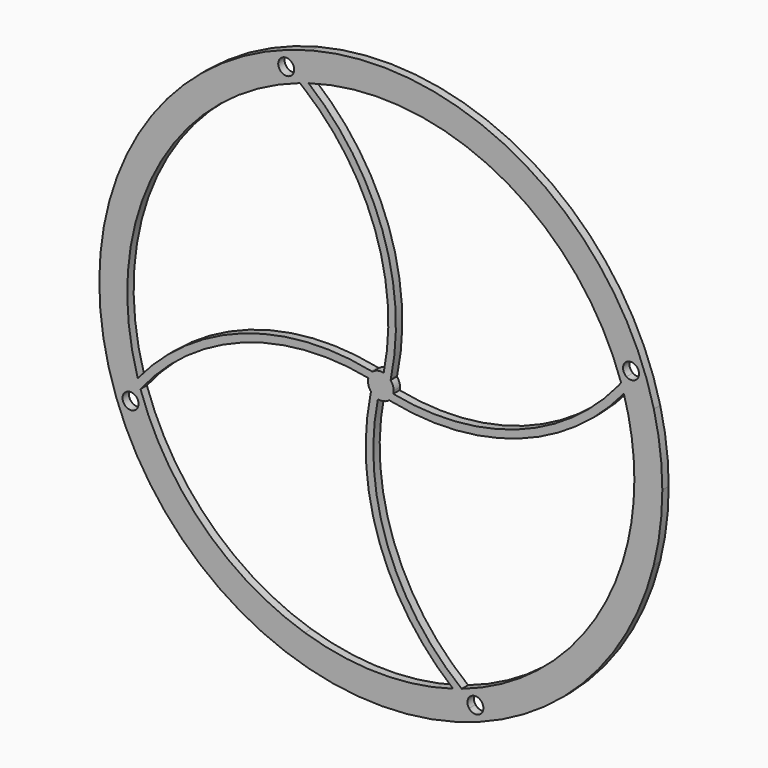
from build123d import *

# Parameters (mm, degrees)
F1_DEPTH = 2


# Not quite as in the source:
# - a feature names something its author has since deleted; it is built from what else it names


with BuildPart() as f1:
    # F0 (on Front) → F1 (new body)
    with BuildSketch(Plane.XZ):
        with BuildLine():
            ThreePointArc((-27.3670955133, 56.9056551345), (-80.5728095325, -11.5155179666), (-27.2210675465, -79.822886236))
            ThreePointArc((-27.2210675465, -79.822886236), (-28.2707166424, -75.9512965825), (-29.0922663621, -72.0249718726))
            ThreePointArc((-29.0922663621, -72.0249718726), (-54.5082769695, -56.802573142), (-70.2520814599, -31.7062061045))
            ThreePointArc((-70.2520814599, -31.7062061045), (-70.6313699985, -32.1947433172), (-71.0054179832, -32.6873044899))
            ThreePointArc((-71.0054179832, -32.6873044899), (-70.0780888504, -33.7565825815), (-69.7442063574, -35.1320161272))
            ThreePointArc((-69.7442063574, -35.1320161272), (-74.7859973818, -37.3299900608), (-72.9649326324, -32.1401471609))
            ThreePointArc((-72.9649326324, -32.1401471609), (-71.9713178078, -30.821081237), (-70.9416554734, -29.5299573821))
            ThreePointArc((-70.9416554734, -29.5299573821), (-66.4396950536, 17.8006515976), (-30.3388328071, 48.7390086816))
            ThreePointArc((-30.3388328071, 48.7390086816), (-30.8273700198, 49.1182972202), (-31.3199311925, 49.4923452049))
            ThreePointArc((-31.3199311925, 49.4923452049), (-36.6541110474, 52.0379628175), (-30.7727738636, 51.4518598542))
            ThreePointArc((-30.7727738636, 51.4518598542), (-29.8904735112, 50.7935939017), (-29.0204405195, 50.1191974536))
            ThreePointArc((-29.0204405195, 50.1191974536), (-28.2798956872, 53.5334090749), (-27.3670955133, 56.9056551345))
        make_face()
        with BuildLine():
            ThreePointArc((-29.0922663621, -72.0249718726), (-28.2707166424, -75.9512965825), (-27.2210675465, -79.822886236))
            ThreePointArc((-27.2210675465, -79.822886236), (26.0907604983, -71.958346724), (58.2730284319, -28.7344688106))
            ThreePointArc((58.2730284319, -28.7344688106), (54.4014575958, -29.7669456779), (50.4763758376, -30.5724283969))
            ThreePointArc((50.4763758376, -30.5724283969), (35.2481065637, -55.9178682056), (10.1931333262, -71.6194547573))
            ThreePointArc((10.1931333262, -71.6194547573), (10.6816705389, -71.9987432958), (11.1742317116, -72.3727912805))
            ThreePointArc((11.1742317116, -72.3727912805), (14.5315947304, -71.2537714989), (16.6189433489, -74.1115796548))
            ThreePointArc((16.6189433489, -74.1115796548), (13.7293813431, -77.1095462072), (10.6270743826, -74.3323059298))
            ThreePointArc((10.6270743826, -74.3323059298), (9.3080084587, -73.3386911051), (8.0168846038, -72.3090287708))
            ThreePointArc((8.0168846038, -72.3090287708), (-10.5589046392, -74.9383627794), (-29.0922663621, -72.0249718726))
        make_face()
        with BuildLine():
            ThreePointArc((58.3098134577, 5.7079947682), (26.0907604983, 49.0779006484), (-27.3670955133, 56.9056551345))
            ThreePointArc((-27.3670955133, 56.9056551345), (-28.2798956872, 53.5334090749), (-29.0204405195, 50.1191974536))
            ThreePointArc((-29.0204405195, 50.1191974536), (-28.589922312, 49.7758651019), (-28.1625840847, 49.4285826951))
            ThreePointArc((-28.1625840847, 49.4285826951), (19.1680248949, 44.9266222753), (50.106381979, 8.8257600288))
            ThreePointArc((50.106381979, 8.8257600288), (50.4856705176, 9.3142972415), (50.8597185023, 9.8068584143))
            ThreePointArc((50.8597185023, 9.8068584143), (51.2230733308, 14.9176875586), (55.5985068765, 12.2515700516))
            ThreePointArc((55.5985068765, 12.2515700516), (54.79648081, 10.2097790271), (52.8192331515, 9.2597010853))
            ThreePointArc((52.8192331515, 9.2597010853), (52.1241754763, 8.329073827), (51.4111721259, 7.4121231804))
            ThreePointArc((51.4111721259, 7.4121231804), (54.8825742735, 6.6494490821), (58.3098134577, 5.7079947682))
        make_face()
        with BuildLine():
            ThreePointArc((50.4763758376, -30.5724283969), (54.4014575958, -29.7669456779), (58.2730284319, -28.7344688106))
            ThreePointArc((58.2730284319, -28.7344688106), (59.886547095, -20.1541655683), (60.4271502595, -11.4402230378))
            ThreePointArc((60.4271502595, -11.4402230378), (59.8958138007, -2.8010030346), (58.3098134577, 5.7079947682))
            ThreePointArc((58.3098134577, 5.7079947682), (54.8825742735, 6.6494490821), (51.4111721259, 7.4121231804))
            ThreePointArc((51.4111721259, 7.4121231804), (51.1051261442, 7.0295570743), (50.7959559925, 6.6495113064))
            ThreePointArc((50.7959559925, 6.6495113064), (52.7659088566, -2.3001782907), (53.4271502595, -11.4402230378))
            ThreePointArc((53.4271502595, -11.4402230378), (52.6851211645, -21.1194320912), (50.4763758376, -30.5724283969))
        make_face()
        with BuildLine():
            ThreePointArc((-12.5201116119, -13.51897209), (-12.5889413468, -13.8437334785), (-12.6559669985, -14.1688719933))
            ThreePointArc((-12.6559669985, -14.1688719933), (-12.4731783685, -13.96568891), (-12.2895816621, -13.7632357104))
            ThreePointArc((-12.2895816621, -13.7632357104), (-12.4080426029, -13.6441201736), (-12.5201116119, -13.51897209))
        make_face()
        with BuildLine():
            ThreePointArc((-12.2895816621, -13.7632357104), (-12.4731783685, -13.96568891), (-12.6559669985, -14.1688719933))
            ThreePointArc((-12.6559669985, -14.1688719933), (-10.3985570941, -46.1115999582), (8.0168846038, -72.3090287708))
            ThreePointArc((8.0168846038, -72.3090287708), (9.1081080721, -71.9740223354), (10.1931333262, -71.6194547573))
            ThreePointArc((10.1931333262, -71.6194547573), (-8.3929341527, -46.0705747238), (-10.7982724135, -14.5681696862))
            ThreePointArc((-10.7982724135, -14.5681696862), (-11.5979884526, -14.2658628235), (-12.2895816621, -13.7632357104))
        make_face()
        with BuildLine():
            ThreePointArc((-70.9416554734, -29.5299573821), (-70.606649038, -30.6211808503), (-70.2520814599, -31.7062061045))
            ThreePointArc((-70.2520814599, -31.7062061045), (-44.7032014264, -13.1201386255), (-13.2007963888, -10.7148003648))
            ThreePointArc((-13.2007963888, -10.7148003648), (-12.862086438, -9.8494851792), (-12.2897757069, -9.1173955477))
            ThreePointArc((-12.2897757069, -9.1173955477), (-12.3762338407, -9.022292149), (-12.4625142647, -8.9270274978))
            ThreePointArc((-12.4625142647, -8.9270274978), (-44.5810834921, -11.0567727884), (-70.9416554734, -29.5299573821))
        make_face()
        with BuildLine():
            ThreePointArc((-71.0054179832, -32.6873044899), (-70.6313699985, -32.1947433172), (-70.2520814599, -31.7062061045))
            ThreePointArc((-70.2520814599, -31.7062061045), (-70.606649038, -30.6211808503), (-70.9416554734, -29.5299573821))
            ThreePointArc((-70.9416554734, -29.5299573821), (-71.9713178078, -30.821081237), (-72.9649326324, -32.1401471609))
            ThreePointArc((-72.9649326324, -32.1401471609), (-71.937377119, -32.2425479097), (-71.0054179832, -32.6873044899))
        make_face()
        with BuildLine():
            ThreePointArc((10.1931333262, -71.6194547573), (9.1081080721, -71.9740223354), (8.0168846038, -72.3090287708))
            ThreePointArc((8.0168846038, -72.3090287708), (9.3080084587, -73.3386911051), (10.6270743826, -74.3323059298))
            ThreePointArc((10.6270743826, -74.3323059298), (10.7294751314, -73.3047504164), (11.1742317116, -72.3727912805))
            ThreePointArc((11.1742317116, -72.3727912805), (10.6816705389, -71.9987432958), (10.1931333262, -71.6194547573))
        make_face()
        with BuildLine():
            ThreePointArc((-28.1625840847, 49.4285826951), (-28.589922312, 49.7758651019), (-29.0204405195, 50.1191974536))
            ThreePointArc((-29.0204405195, 50.1191974536), (-29.1146314874, 49.6144442417), (-29.2050550996, 49.1090025402))
            ThreePointArc((-29.2050550996, 49.1090025402), (-28.6845055424, 49.2710301885), (-28.1625840847, 49.4285826951))
        make_face()
        with BuildLine():
            ThreePointArc((-29.2050550996, 49.1090025402), (-29.1146314874, 49.6144442417), (-29.0204405195, 50.1191974536))
            ThreePointArc((-29.0204405195, 50.1191974536), (-29.8904735112, 50.7935939017), (-30.7727738636, 51.4518598542))
            ThreePointArc((-30.7727738636, 51.4518598542), (-30.7666762774, 51.3415715733), (-30.7646428299, 51.2311335791))
            ThreePointArc((-30.7646428299, 51.2311335791), (-30.9068346739, 50.3184821977), (-31.3199311925, 49.4923452049))
            ThreePointArc((-31.3199311925, 49.4923452049), (-30.8273700198, 49.1182972202), (-30.3388328071, 48.7390086816))
            ThreePointArc((-30.3388328071, 48.7390086816), (-29.7728126001, 48.9266674182), (-29.2050550996, 49.1090025402))
        make_face()
        with BuildLine():
            ThreePointArc((50.7959559925, 6.6495113064), (51.1051261442, 7.0295570743), (51.4111721259, 7.4121231804))
            ThreePointArc((51.4111721259, 7.4121231804), (50.9618140768, 7.4971572567), (50.5118990943, 7.5791935838))
            ThreePointArc((50.5118990943, 7.5791935838), (50.6557066113, 7.1148960249), (50.7959559925, 6.6495113064))
        make_face()
        with BuildLine():
            ThreePointArc((50.5118990943, 7.5791935838), (50.9618140768, 7.4971572567), (51.4111721259, 7.4121231804))
            ThreePointArc((51.4111721259, 7.4121231804), (52.1241754763, 8.329073827), (52.8192331515, 9.2597010853))
            ThreePointArc((52.8192331515, 9.2597010853), (51.7916776381, 9.362101834), (50.8597185023, 9.8068584143))
            ThreePointArc((50.8597185023, 9.8068584143), (50.4856705176, 9.3142972415), (50.106381979, 8.8257600288))
            ThreePointArc((50.106381979, 8.8257600288), (50.3123573205, 8.2035232495), (50.5118990943, 7.5791935838))
        make_face()
        with BuildLine():
            ThreePointArc((-12.5201116119, -13.51897209), (-12.4080426029, -13.6441201736), (-12.2895816621, -13.7632357104))
            ThreePointArc((-12.2895816621, -13.7632357104), (-11.1948099524, -12.5887570771), (-10.0728497405, -11.4402230378))
            ThreePointArc((-10.0728497405, -11.4402230378), (-10.9940718567, -11.2075300608), (-11.9189886514, -10.9899866588))
            ThreePointArc((-11.9189886514, -10.9899866588), (-12.2332943861, -12.2512124569), (-12.5201116119, -13.51897209))
        make_face()
        with BuildLine():
            ThreePointArc((-10.0728497405, -11.4402230378), (-11.1948099524, -12.5887570771), (-12.2895816621, -13.7632357104))
            ThreePointArc((-12.2895816621, -13.7632357104), (-11.5979884526, -14.2658628235), (-10.7982724135, -14.5681696862))
            ThreePointArc((-10.7982724135, -14.5681696862), (-10.6643076305, -13.9264868582), (-10.5230861195, -13.2863619488))
            ThreePointArc((-10.5230861195, -13.2863619488), (-10.5381735464, -13.2824253135), (-10.5532599463, -13.2784847442))
            Line((-10.5532599463, -13.2784847442), (-10.0728497405, -11.4402230378))
        make_face()
        with BuildLine():
            ThreePointArc((-13.2007963888, -10.7148003648), (-13.1931994446, -12.1976568722), (-12.5201116119, -13.51897209))
            ThreePointArc((-12.5201116119, -13.51897209), (-12.2332943861, -12.2512124569), (-11.9189886514, -10.9899866588))
            ThreePointArc((-11.9189886514, -10.9899866588), (-12.5591135608, -10.8487651478), (-13.2007963888, -10.7148003648))
        make_face()
        with BuildLine():
            ThreePointArc((-12.2897757069, -9.1173955477), (-12.862086438, -9.8494851792), (-13.2007963888, -10.7148003648))
            ThreePointArc((-13.2007963888, -10.7148003648), (-12.5591135608, -10.8487651478), (-11.9189886514, -10.9899866588))
            ThreePointArc((-11.9189886514, -10.9899866588), (-11.9150520162, -10.9748992319), (-11.9111114468, -10.9598128319))
            Line((-11.9111114468, -10.9598128319), (-10.0728497405, -11.4402230378))
            ThreePointArc((-10.0728497405, -11.4402230378), (-11.1948573752, -10.2917364213), (-12.2897757069, -9.1173955477))
        make_face()
        with BuildLine():
            ThreePointArc((-69.7442063574, -35.1320161272), (-70.0780888504, -33.7565825815), (-71.0054179832, -32.6873044899))
            ThreePointArc((-71.0054179832, -32.6873044899), (-71.3040153489, -33.088497971), (-71.5991359801, -33.4922558304))
            ThreePointArc((-71.5991359801, -33.4922558304), (-70.9707717301, -34.2073920832), (-70.7442063574, -35.1320161272))
            ThreePointArc((-70.7442063574, -35.1320161272), (-73.6278272269, -36.9262329923), (-73.9634205165, -33.5466086609))
            ThreePointArc((-73.9634205165, -33.5466086609), (-73.469248174, -32.839777435), (-72.9649326324, -32.1401471609))
            ThreePointArc((-72.9649326324, -32.1401471609), (-74.7859973818, -37.3299900608), (-69.7442063574, -35.1320161272))
        make_face()
        with BuildLine():
            ThreePointArc((-71.5991359801, -33.4922558304), (-71.3040153489, -33.088497971), (-71.0054179832, -32.6873044899))
            ThreePointArc((-71.0054179832, -32.6873044899), (-71.937377119, -32.2425479097), (-72.9649326324, -32.1401471609))
            ThreePointArc((-72.9649326324, -32.1401471609), (-73.469248174, -32.839777435), (-73.9634205165, -33.5466086609))
            ThreePointArc((-73.9634205165, -33.5466086609), (-72.7901724606, -33.1325444177), (-71.5991359801, -33.4922558304))
        make_face()
        with BuildLine():
            ThreePointArc((11.1742317116, -72.3727912805), (10.7294751314, -73.3047504164), (10.6270743826, -74.3323059298))
            ThreePointArc((10.6270743826, -74.3323059298), (11.3267046567, -74.8366214714), (12.0335358826, -75.3307938138))
            ThreePointArc((12.0335358826, -75.3307938138), (11.6194716394, -74.1575457579), (11.9791830521, -72.9665092775))
            ThreePointArc((11.9791830521, -72.9665092775), (11.5754251927, -72.6713886463), (11.1742317116, -72.3727912805))
        make_face()
        with BuildLine():
            ThreePointArc((12.0335358826, -75.3307938138), (11.3267046567, -74.8366214714), (10.6270743826, -74.3323059298))
            ThreePointArc((10.6270743826, -74.3323059298), (13.7293813431, -77.1095462072), (16.6189433489, -74.1115796548))
            ThreePointArc((16.6189433489, -74.1115796548), (14.5315947304, -71.2537714989), (11.1742317116, -72.3727912805))
            ThreePointArc((11.1742317116, -72.3727912805), (11.5754251927, -72.6713886463), (11.9791830521, -72.9665092775))
            ThreePointArc((11.9791830521, -72.9665092775), (14.2191430683, -72.2037640723), (15.6189433489, -74.1115796548))
            ThreePointArc((15.6189433489, -74.1115796548), (14.2628319524, -76.0050968758), (12.0335358826, -75.3307938138))
        make_face()
        with BuildLine():
            ThreePointArc((-28.1625840847, 49.4285826951), (-28.6845055424, 49.2710301885), (-29.2050550996, 49.1090025402))
            ThreePointArc((-29.2050550996, 49.1090025402), (-29.3013575877, 48.545087408), (-29.3929706411, 47.9803914774))
            ThreePointArc((-29.3929706411, 47.9803914774), (-11.5464019221, 22.6200733478), (-9.3474270674, -8.3122763895))
            ThreePointArc((-9.3474270674, -8.3122763895), (-8.4819953839, -8.6510527838), (-7.7498370678, -9.2234911162))
            ThreePointArc((-7.7498370678, -9.2234911162), (-7.6548806672, -9.1371958925), (-7.5597630163, -9.051078437))
            ThreePointArc((-7.5597630163, -9.051078437), (-9.6893112365, 23.0677602114), (-28.1625840847, 49.4285826951))
        make_face()
        with BuildLine():
            ThreePointArc((-29.3929706411, 47.9803914774), (-29.3013575877, 48.545087408), (-29.2050550996, 49.1090025402))
            ThreePointArc((-29.2050550996, 49.1090025402), (-29.7728126001, 48.9266674182), (-30.3388328071, 48.7390086816))
            ThreePointArc((-30.3388328071, 48.7390086816), (-29.8639157079, 48.3621762923), (-29.3929706411, 47.9803914774))
        make_face()
        with BuildLine():
            ThreePointArc((-30.7646428299, 51.2311335791), (-30.7666762774, 51.3415715733), (-30.7727738636, 51.4518598542))
            ThreePointArc((-30.7727738636, 51.4518598542), (-31.4724041376, 51.9561753958), (-32.1792353635, 52.4503477382))
            ThreePointArc((-32.1792353635, 52.4503477382), (-31.8711256088, 51.8750221826), (-31.7646428299, 51.2311335791))
            ThreePointArc((-31.7646428299, 51.2311335791), (-31.8568272474, 50.6309338597), (-32.124882533, 50.0860632018))
            ThreePointArc((-32.124882533, 50.0860632018), (-31.7211246736, 49.7909425706), (-31.3199311925, 49.4923452049))
            ThreePointArc((-31.3199311925, 49.4923452049), (-30.9068346739, 50.3184821977), (-30.7646428299, 51.2311335791))
        make_face()
        with BuildLine():
            ThreePointArc((-32.1792353635, 52.4503477382), (-31.4724041376, 51.9561753958), (-30.7727738636, 51.4518598542))
            ThreePointArc((-30.7727738636, 51.4518598542), (-36.6541110474, 52.0379628175), (-31.3199311925, 49.4923452049))
            ThreePointArc((-31.3199311925, 49.4923452049), (-31.7211246736, 49.7909425706), (-32.124882533, 50.0860632018))
            ThreePointArc((-32.124882533, 50.0860632018), (-35.7641145394, 51.185167476), (-32.1792353635, 52.4503477382))
        make_face()
        with BuildLine():
            ThreePointArc((-7.9941006882, -13.8874849093), (-7.6696946098, -13.9562403689), (-7.3449122183, -14.0231956907))
            ThreePointArc((-7.3449122183, -14.0231956907), (-7.5478301275, -13.8405739674), (-7.7500222504, -13.6571490043))
            ThreePointArc((-7.7500222504, -13.6571490043), (-7.8690501416, -13.7755079493), (-7.9941006882, -13.8874849093))
        make_face()
        with BuildLine():
            ThreePointArc((-7.7500222504, -13.6571490043), (-7.5478301275, -13.8405739674), (-7.3449122183, -14.0231956907))
            ThreePointArc((-7.3449122183, -14.0231956907), (24.5981851662, -11.7660519999), (50.7959559925, 6.6495113064))
            ThreePointArc((50.7959559925, 6.6495113064), (50.6557066113, 7.1148960249), (50.5118990943, 7.5791935838))
            ThreePointArc((50.5118990943, 7.5791935838), (49.8930363162, 7.6869831447), (49.2732124019, 7.7891009341))
            ThreePointArc((49.2732124019, 7.7891009341), (23.9320992091, -9.9863481746), (-6.9449030921, -12.1656457109))
            ThreePointArc((-6.9449030921, -12.1656457109), (-7.2472736584, -12.9654797683), (-7.7500222504, -13.6571490043))
        make_face()
        with BuildLine():
            ThreePointArc((49.2732124019, 7.7891009341), (49.8930363162, 7.6869831447), (50.5118990943, 7.5791935838))
            ThreePointArc((50.5118990943, 7.5791935838), (50.3123573205, 8.2035232495), (50.106381979, 8.8257600288))
            ThreePointArc((50.106381979, 8.8257600288), (49.6927740639, 8.3050379491), (49.2732124019, 7.7891009341))
        make_face()
        with BuildLine():
            ThreePointArc((50.8597185023, 9.8068584143), (51.7916776381, 9.362101834), (52.8192331515, 9.2597010853))
            ThreePointArc((52.8192331515, 9.2597010853), (53.0275327482, 9.5460981807), (53.2341325227, 9.8337238948))
            ThreePointArc((53.2341325227, 9.8337238948), (52.1548181767, 9.7912569947), (51.1583297131, 10.2080706662))
            ThreePointArc((51.1583297131, 10.2080706662), (51.0094573534, 10.0071420874), (50.8597185023, 9.8068584143))
        make_face()
        with BuildLine():
            ThreePointArc((53.2341325227, 9.8337238948), (53.0275327482, 9.5460981807), (52.8192331515, 9.2597010853))
            ThreePointArc((52.8192331515, 9.2597010853), (54.79648081, 10.2097790271), (55.5985068765, 12.2515700516))
            ThreePointArc((55.5985068765, 12.2515700516), (51.2230733308, 14.9176875586), (50.8597185023, 9.8068584143))
            ThreePointArc((50.8597185023, 9.8068584143), (51.0094573534, 10.0071420874), (51.1583297131, 10.2080706662))
            ThreePointArc((51.1583297131, 10.2080706662), (51.4475166308, 14.4708540474), (55.0985068765, 12.2515700516))
            ThreePointArc((55.0985068765, 12.2515700516), (54.578287687, 10.7249830274), (53.2341325227, 9.8337238948))
        make_face()
        with BuildLine():
            Line((-9.5924395346, -9.6019613315), (-10.0728497405, -11.4402230378))
            ThreePointArc((-10.0728497405, -11.4402230378), (-8.9243157011, -10.3182628259), (-7.7498370678, -9.2234911162))
            ThreePointArc((-7.7498370678, -9.2234911162), (-8.4819953839, -8.6510527838), (-9.3474270674, -8.3122763895))
            ThreePointArc((-9.3474270674, -8.3122763895), (-9.4813918505, -8.9539592174), (-9.6226133615, -9.5940841269))
            ThreePointArc((-9.6226133615, -9.5940841269), (-9.6075259345, -9.5980207621), (-9.5924395346, -9.6019613315))
        make_face()
        with BuildLine():
            Line((-8.2345880341, -11.9206332437), (-10.0728497405, -11.4402230378))
            ThreePointArc((-10.0728497405, -11.4402230378), (-8.924363124, -12.5622306726), (-7.7500222504, -13.6571490043))
            ThreePointArc((-7.7500222504, -13.6571490043), (-7.2472736584, -12.9654797683), (-6.9449030921, -12.1656457109))
            ThreePointArc((-6.9449030921, -12.1656457109), (-7.5865859201, -12.0316809278), (-8.2267108295, -11.8904594168))
            ThreePointArc((-8.2267108295, -11.8904594168), (-8.2306474647, -11.9055468438), (-8.2345880341, -11.9206332437))
        make_face()
        with BuildLine():
            ThreePointArc((-7.7498370678, -9.2234911162), (-8.9243157011, -10.3182628259), (-10.0728497405, -11.4402230378))
            ThreePointArc((-10.0728497405, -11.4402230378), (-9.1516276243, -11.6729160149), (-8.2267108295, -11.8904594168))
            ThreePointArc((-8.2267108295, -11.8904594168), (-7.9124050948, -10.6292336188), (-7.625587869, -9.3614739856))
            ThreePointArc((-7.625587869, -9.3614739856), (-7.686714869, -9.2915842443), (-7.7498370678, -9.2234911162))
        make_face()
        with BuildLine():
            ThreePointArc((-10.5230861195, -13.2863619488), (-10.3055427175, -12.361445154), (-10.0728497405, -11.4402230378))
            Line((-10.0728497405, -11.4402230378), (-10.5532599463, -13.2784847442))
            ThreePointArc((-10.5532599463, -13.2784847442), (-10.5381735464, -13.2824253135), (-10.5230861195, -13.2863619488))
        make_face()
        with BuildLine():
            ThreePointArc((-12.2897757069, -9.1173955477), (-11.1948573752, -10.2917364213), (-10.0728497405, -11.4402230378))
            ThreePointArc((-10.0728497405, -11.4402230378), (-9.8401567634, -10.5190009216), (-9.6226133615, -9.5940841269))
            ThreePointArc((-9.6226133615, -9.5940841269), (-10.8838391595, -9.2797783922), (-12.1515987927, -8.9929611664))
            ThreePointArc((-12.1515987927, -8.9929611664), (-12.2215881949, -9.0541779116), (-12.2897757069, -9.1173955477))
        make_face()
        with BuildLine():
            ThreePointArc((-8.2267108295, -11.8904594168), (-9.1516276243, -11.6729160149), (-10.0728497405, -11.4402230378))
            Line((-10.0728497405, -11.4402230378), (-8.2345880341, -11.9206332437))
            ThreePointArc((-8.2345880341, -11.9206332437), (-8.2306474647, -11.9055468438), (-8.2267108295, -11.8904594168))
        make_face()
        with BuildLine():
            ThreePointArc((-9.6226133615, -9.5940841269), (-9.8401567634, -10.5190009216), (-10.0728497405, -11.4402230378))
            Line((-10.0728497405, -11.4402230378), (-9.5924395346, -9.6019613315))
            ThreePointArc((-9.5924395346, -9.6019613315), (-9.6075259345, -9.5980207621), (-9.6226133615, -9.5940841269))
        make_face()
        with BuildLine():
            ThreePointArc((-7.7500222504, -13.6571490043), (-8.924363124, -12.5622306726), (-10.0728497405, -11.4402230378))
            ThreePointArc((-10.0728497405, -11.4402230378), (-10.3055427175, -12.361445154), (-10.5230861195, -13.2863619488))
            ThreePointArc((-10.5230861195, -13.2863619488), (-9.2618603214, -13.6006676835), (-7.9941006882, -13.8874849093))
            ThreePointArc((-7.9941006882, -13.8874849093), (-7.8690501416, -13.7755079493), (-7.7500222504, -13.6571490043))
        make_face()
        with BuildLine():
            ThreePointArc((-11.9189886514, -10.9899866588), (-10.9940718567, -11.2075300608), (-10.0728497405, -11.4402230378))
            Line((-10.0728497405, -11.4402230378), (-11.9111114468, -10.9598128319))
            ThreePointArc((-11.9111114468, -10.9598128319), (-11.9150520162, -10.9748992319), (-11.9189886514, -10.9899866588))
        make_face()
        with BuildLine():
            ThreePointArc((-10.5230861195, -13.2863619488), (-10.6643076305, -13.9264868582), (-10.7982724135, -14.5681696862))
            ThreePointArc((-10.7982724135, -14.5681696862), (-9.3154159061, -14.560572742), (-7.9941006882, -13.8874849093))
            ThreePointArc((-7.9941006882, -13.8874849093), (-9.2618603214, -13.6006676835), (-10.5230861195, -13.2863619488))
        make_face()
        with BuildLine():
            ThreePointArc((-12.4625142647, -8.9270274978), (-12.3762338407, -9.022292149), (-12.2897757069, -9.1173955477))
            ThreePointArc((-12.2897757069, -9.1173955477), (-12.2215881949, -9.0541779116), (-12.1515987927, -8.9929611664))
            ThreePointArc((-12.1515987927, -8.9929611664), (-12.3070127215, -8.9597877558), (-12.4625142647, -8.9270274978))
        make_face()
        with BuildLine():
            ThreePointArc((-7.625587869, -9.3614739856), (-7.5924695565, -9.2063198731), (-7.5597630163, -9.051078437))
            ThreePointArc((-7.5597630163, -9.051078437), (-7.6548806672, -9.1371958925), (-7.7498370678, -9.2234911162))
            ThreePointArc((-7.7498370678, -9.2234911162), (-7.686714869, -9.2915842443), (-7.625587869, -9.3614739856))
        make_face()
        with BuildLine():
            ThreePointArc((53.8177210355, 10.6661625852), (53.5276959283, 10.2487029623), (53.2341325227, 9.8337238948))
            ThreePointArc((53.2341325227, 9.8337238948), (54.578287687, 10.7249830274), (55.0985068765, 12.2515700516))
            ThreePointArc((55.0985068765, 12.2515700516), (51.4475166308, 14.4708540474), (51.1583297131, 10.2080706662))
            ThreePointArc((51.1583297131, 10.2080706662), (51.3063190398, 10.4096215716), (51.4534364992, 10.6118097547))
            ThreePointArc((51.4534364992, 10.6118097547), (51.6738828325, 14.0250046789), (54.5985068765, 12.2515700516))
            ThreePointArc((54.5985068765, 12.2515700516), (54.3927237416, 11.3679491821), (53.8177210355, 10.6661625852))
        make_face()
        with BuildLine():
            ThreePointArc((51.1583297131, 10.2080706662), (52.1548181767, 9.7912569947), (53.2341325227, 9.8337238948))
            ThreePointArc((53.2341325227, 9.8337238948), (53.5276959283, 10.2487029623), (53.8177210355, 10.6661625852))
            ThreePointArc((53.8177210355, 10.6661625852), (52.6444729797, 10.252098342), (51.4534364992, 10.6118097547))
            ThreePointArc((51.4534364992, 10.6118097547), (51.3063190398, 10.4096215716), (51.1583297131, 10.2080706662))
        make_face()
        with BuildLine():
            ThreePointArc((-7.625587869, -9.3614739856), (-7.9124050948, -10.6292336188), (-8.2267108295, -11.8904594168))
            ThreePointArc((-8.2267108295, -11.8904594168), (-7.5865859201, -12.0316809278), (-6.9449030921, -12.1656457109))
            ThreePointArc((-6.9449030921, -12.1656457109), (-6.8827077662, -11.8053017608), (-6.8618859771, -11.4402230378))
            ThreePointArc((-6.8618859771, -11.4402230378), (-7.0588526039, -10.3329247264), (-7.625587869, -9.3614739856))
        make_face()
        with BuildLine():
            ThreePointArc((-12.1515987927, -8.9929611664), (-10.8838391595, -9.2797783922), (-9.6226133615, -9.5940841269))
            ThreePointArc((-9.6226133615, -9.5940841269), (-9.4813918505, -8.9539592174), (-9.3474270674, -8.3122763895))
            ThreePointArc((-9.3474270674, -8.3122763895), (-10.8302835749, -8.3198733337), (-12.1515987927, -8.9929611664))
        make_face()
    extrude(amount=F1_DEPTH)


solid = f1.part
